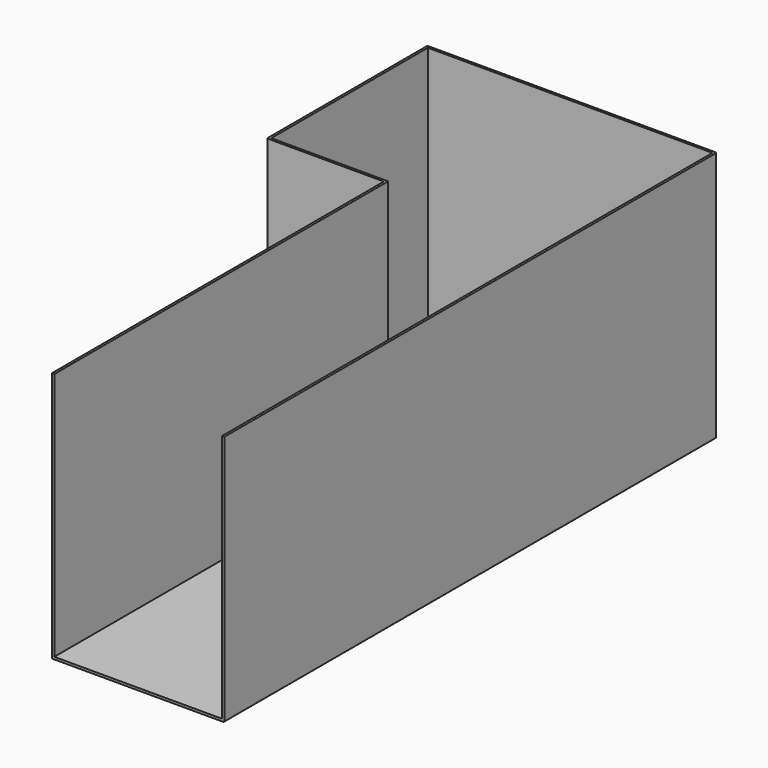
from build123d import *

# Parameters (mm, degrees)
F1_DEPTH = 426
F3_DEPTH = 4
F4_R     = 2


# Not quite as in the source:
# - a feature names something its author has since deleted; it is built from what else it names


with BuildPart() as f1:
    # F0 (on Top) → F1 (new body)
    with BuildSketch(Plane.XY):
        Polygon((495, 0), (0, 0), (0, -343), (200, -343), (200, -1053), (204, -1053), (204, -339), (4, -339), (4, -4), (491, -4), (491, -1053), (495, -1053), align=None)
    extrude(amount=F1_DEPTH)

    # F2 (on Top) → F3 (join)
    with BuildSketch(Plane.XY):
        Polygon((0, -343), (200, -343), (199.9874711037, -1053), (495, -1053), (495, 0), (0, 0), align=None)
    extrude(amount=-F3_DEPTH)

    # F4
    f4_edges = [f1.edges().sort_by_distance(p)[0] for p in [
        (100, -343, -4),
        (0, -171.5, -4),
        (247.5, 0, -4),
        (0, -343, 211),
        (0, 0, 211),
        (495, 0, 211),
        (199.993736, -698, -4),
        (495, -526.5, -4),
    ]]
    fillet(f4_edges, radius=F4_R)


solid = f1.part
